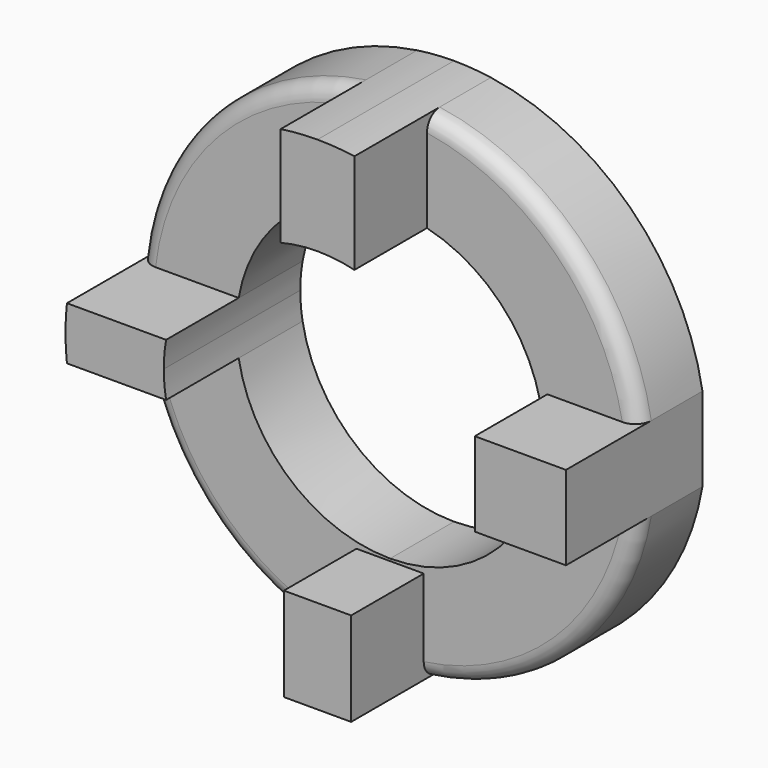
from build123d import *

# Parameters (mm, degrees)
F1_DEPTH = 25.4
F2_DEPTH = 54.2429313064
F0_W     = 28.9929530091
F0_H     = 13.3561033948
F0_W_2   = 10.6932765457
F0_H_2   = 29.8016675711
F3_R     = 5.08
F3_2_R   = 5.08


with BuildPart() as f1:
    # F0 (on Front) → F1 (new body)
    with BuildSketch(Plane.XZ):
        with BuildLine():
            ThreePointArc((11.7221610006, 47.4434716165), (38.4782788305, 30.1282942728), (48.8701550801, 0))
            Line((48.8701550801, 0), (49.9914412338, 0))
            Line((49.9914412338, 0), (49.9914412338, 13.3561033948))
            Line((49.9914412338, 13.3561033948), (78.9843942429, 13.3561033948))
            ThreePointArc((78.9843942429, 13.3561033948), (56.055353156, 57.2251466959), (11.7221610006, 79.2433654844))
            Line((11.7221610006, 79.2433654844), (11.7221610006, 47.4434716165))
        make_face()
        with BuildLine():
            Line((49.9914412338, 0), (48.8701550801, 0))
            ThreePointArc((48.8701550801, 0), (34.5564180548, -34.5564180548), (0, -48.8701550801))
            Line((0, -48.8701550801), (0, -49.5870839528))
            Line((0, -49.5870839528), (10.6932765457, -49.5870839528))
            Line((10.6932765457, -49.5870839528), (10.6932765457, -79.3887515239))
            ThreePointArc((10.6932765457, -79.3887515239), (55.6830208794, -57.5875092148), (78.9843942429, -13.3561033948))
            Line((78.9843942429, -13.3561033948), (49.9914412338, -13.3561033948))
            Line((49.9914412338, -13.3561033948), (49.9914412338, 0))
        make_face()
        with BuildLine():
            Line((0, -49.5870839528), (0, -48.8701550801))
            ThreePointArc((0, -48.8701550801), (-31.4400806584, -37.4140800468), (-48.1398797488, -8.4168898844))
            Line((-48.1398797488, -8.4168898844), (-79.6622620598, -8.4168898844))
            ThreePointArc((-79.6622620598, -8.4168898844), (-57.4480819986, -55.8268564984), (-10.6932765457, -79.3887515239))
            Line((-10.6932765457, -79.3887515239), (-10.6932765457, -49.5870839528))
            Line((-10.6932765457, -49.5870839528), (0, -49.5870839528))
        make_face()
    extrude(amount=F1_DEPTH)

    # F3
    f3_edges = [f1.edges().sort_by_distance(p)[0] for p in [
        (-57.448082, -25.4, -55.826856),
        (56.055353, -25.4, 57.225147),
        (55.683021, -25.4, -57.587509),
    ]]
    fillet(f3_edges, radius=F3_R)


with BuildPart() as f1b:
    # F0 (on Front) → F1, piece 2 (new body)
    with BuildSketch(Plane.XZ):
        with BuildLine():
            ThreePointArc((-48.1398797488, 8.4168898844), (-35.7300224054, 33.341529006), (-11.7221610006, 47.4434716165))
            Line((-11.7221610006, 47.4434716165), (-11.7221610006, 79.2433654844))
            ThreePointArc((-11.7221610006, 79.2433654844), (-57.8089578353, 55.4530831047), (-79.6622620598, 8.4168898844))
            Line((-79.6622620598, 8.4168898844), (-48.1398797488, 8.4168898844))
        make_face()
    extrude(amount=F1_DEPTH)

    # F3#2
    f3_2_edges = [f1b.edges().sort_by_distance(p)[0] for p in [
        (-57.808958, -25.4, 55.453083),
    ]]
    fillet(f3_2_edges, radius=F3_2_R)


with BuildPart() as f2:
    # F0 (on Front) → F2 (new body)
    with BuildSketch(Plane.XZ):
        with BuildLine():
            ThreePointArc((0, 48.8701550801), (5.9043307036, 48.5121730754), (11.7221610006, 47.4434716165))
            Line((11.7221610006, 47.4434716165), (11.7221610006, 79.2433654844))
            ThreePointArc((11.7221610006, 79.2433654844), (5.8769176771, 79.8898108048), (0, 80.1056803967))
            Line((0, 80.1056803967), (0, 48.8701550801))
        make_face()
        with BuildLine():
            ThreePointArc((-11.7221610006, 47.4434716165), (-5.9043307036, 48.5121730754), (0, 48.8701550801))
            Line((0, 48.8701550801), (0, 80.1056803967))
            ThreePointArc((0, 80.1056803967), (-5.8769176771, 79.8898108048), (-11.7221610006, 79.2433654844))
            Line((-11.7221610006, 79.2433654844), (-11.7221610006, 47.4434716165))
        make_face()
    extrude(amount=F2_DEPTH)


with BuildPart() as f2b:
    # F0 (on Front) → F2, piece 2 (new body)
    with BuildSketch(Plane.XZ):
        with Locations((64.4879177384, -6.6780516974)):
            Rectangle(F0_W, F0_H)
        with Locations((64.4879177384, 6.6780516974)):
            Rectangle(F0_W, F0_H)
    extrude(amount=F2_DEPTH)


with BuildPart() as f2c:
    # F0 (on Front) → F2, piece 3 (new body)
    with BuildSketch(Plane.XZ):
        with BuildLine():
            Line((-79.6622620598, -8.4168898844), (-48.1398797488, -8.4168898844))
            ThreePointArc((-48.1398797488, -8.4168898844), (-48.6872439475, -4.2242554783), (-48.8701550801, 0))
            Line((-48.8701550801, 0), (-80.1056803967, 0))
            ThreePointArc((-80.1056803967, 0), (-79.9947490028, -4.2142809335), (-79.6622620598, -8.4168898844))
        make_face()
        with BuildLine():
            ThreePointArc((-48.8701550801, 0), (-48.6872439475, 4.2242554783), (-48.1398797488, 8.4168898844))
            Line((-48.1398797488, 8.4168898844), (-79.6622620598, 8.4168898844))
            ThreePointArc((-79.6622620598, 8.4168898844), (-79.9947490028, 4.2142809335), (-80.1056803967, 0))
            Line((-80.1056803967, 0), (-48.8701550801, 0))
        make_face()
    extrude(amount=F2_DEPTH)


with BuildPart() as f2d:
    # F0 (on Front) → F2, piece 4 (new body)
    with BuildSketch(Plane.XZ):
        with Locations((5.3466382728, -64.4879177384)):
            Rectangle(F0_W_2, F0_H_2)
        with Locations((-5.3466382728, -64.4879177384)):
            Rectangle(F0_W_2, F0_H_2)
    extrude(amount=F2_DEPTH)


solid = Compound([f1.part, f1b.part, f2.part, f2b.part, f2c.part, f2d.part])
